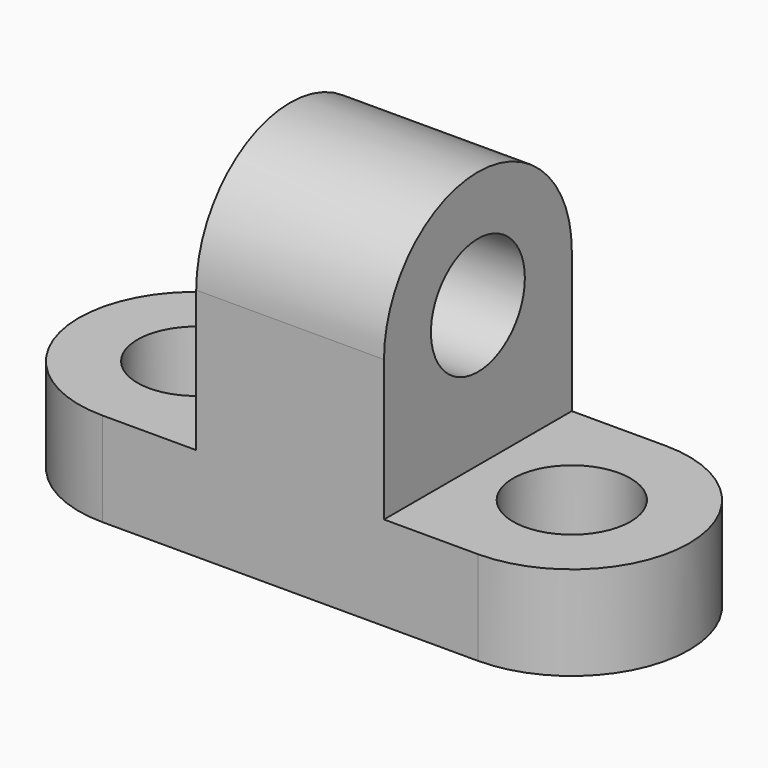
from build123d import *

# Parameters (mm, degrees)
F1_R     = 12.5
F2_DEPTH = 20
F3_DEPTH = 50
F4_DEPTH = 25
F6_DEPTH = 40
F7_DEPTH = 40


with BuildPart() as f2:
    # F1 (on Top) → F2 (new body)
    with BuildSketch(Plane.XY):
        with BuildLine():
            Line((80, 0), (0, 0))
            ThreePointArc((0, 0), (-25, -25), (0, -50))
            Line((0, -50), (80, -50))
            ThreePointArc((80, -50), (105, -25), (80, 0))
        make_face()
        with Locations((0, -25)):
            Circle(F1_R, mode=Mode.SUBTRACT)
        with Locations((80, -25)):
            Circle(F1_R, mode=Mode.SUBTRACT)
    extrude(amount=F2_DEPTH)

    # F0 (on Front) → F3 (join)
    with BuildSketch(Plane.XZ):
        Polygon((0, 20), (0, 0), (80, 0), (80, 19.3890032326), (60, 19.3890032326), (60, 50), (20, 50), (20, 20), align=None)
    extrude(amount=F3_DEPTH)

    # F1 (on Top) → F4 (cut)
    with BuildSketch(Plane.XY):
        with Locations((0, -25)):
            Circle(F1_R)
        with Locations((80, -25)):
            Circle(F1_R)
    extrude(amount=F4_DEPTH, mode=Mode.SUBTRACT)

    # F5 (on face) → F6 (join)
    with BuildSketch(Plane(origin=(20, 0, 0), x_dir=(0, -1, 0), z_dir=(-1, 0, 0))):
        with BuildLine():
            ThreePointArc((12.5, 50), (25, 62.5), (37.5, 50))
            Line((37.5, 50), (50, 50))
            ThreePointArc((50, 50), (25, 75), (0, 50))
            Line((0, 50), (12.5, 50))
        make_face()
    extrude(amount=-F6_DEPTH)

    # F5 (on face) → F7 (cut)
    with BuildSketch(Plane(origin=(20, 0, 0), x_dir=(0, -1, 0), z_dir=(-1, 0, 0))):
        with BuildLine():
            ThreePointArc((12.5, 50), (25, 37.5), (37.5, 50))
            Line((37.5, 50), (12.5, 50))
        make_face()
    extrude(amount=-F7_DEPTH, mode=Mode.SUBTRACT)


solid = f2.part
